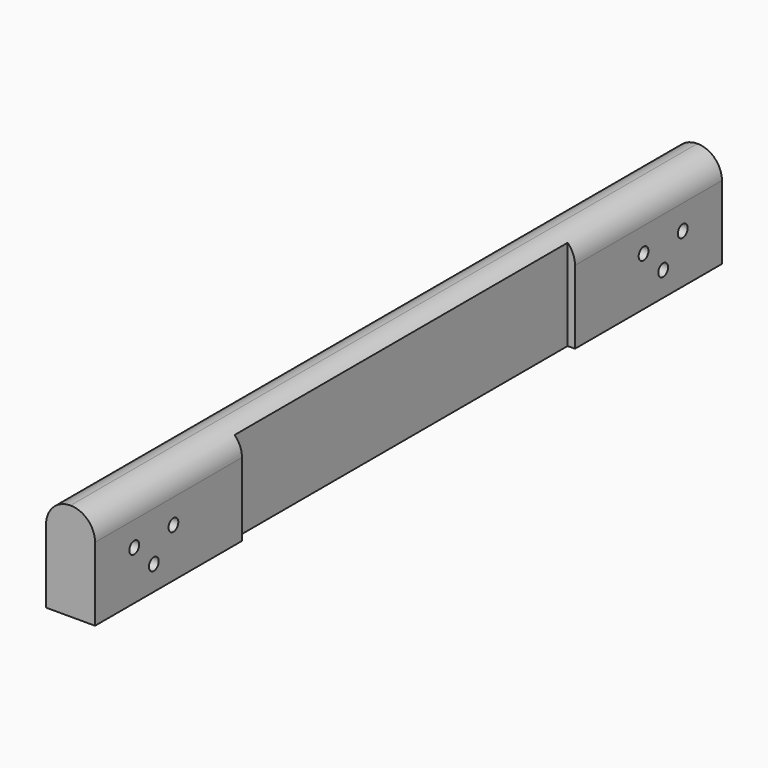
from build123d import *

# Parameters (mm, degrees)
F0_W     = 12.7
F0_H     = 25.4
F1_DEPTH = 101.6
F2_R     = 6.34999
F3_R     = 1.5875
F4_DEPTH = 25.4
F5_W     = 3.81
F5_H     = 107.95
F6_DEPTH = 25.4


# Not quite as in the source:
# - a fillet or chamfer is up to 0.001 mm smaller than in the source, because OpenCascade refuses the exact size


with BuildPart() as f1:
    # F0 (on Front) → F1 (new body, symmetric)
    with BuildSketch(Plane.XZ):
        Rectangle(F0_W, F0_H)
    extrude(amount=F1_DEPTH, both=True)

    # F2 (radius 6.35 in the source; OpenCascade refuses exactly that, so slightly less here)
    f2_edges = [f1.edges().sort_by_distance(p)[0] for p in [
        (-6.35, 0, 12.7),
        (6.35, 0, 12.7),
    ]]
    fillet(f2_edges, radius=F2_R)

    # F3 (on face) → F4 (cut)
    with BuildSketch(Plane(origin=(-6.35, 0, 0), x_dir=(0, -1, 0), z_dir=(-1, 0, 0))):
        with BuildLine():
            Line((-77.7875, 0), (-74.6125, 0))
            ThreePointArc((-74.6125, 0), (-76.2, 1.5875), (-77.7875, 0))
        make_face()
        with Locations((-88.9, 0)):
            Circle(F3_R)
        with BuildLine():
            ThreePointArc((90.4875, 0), (88.9, 1.5875), (87.3125, 0))
            ThreePointArc((87.3125, 0), (88.9, -1.5875), (90.4875, 0))
        make_face()
        with BuildLine():
            ThreePointArc((77.7875, 0), (76.2, 1.5875), (74.6125, 0))
            Line((74.6125, 0), (77.7875, 0))
        make_face()
        with BuildLine():
            Line((77.7875, 0), (74.6125, 0))
            ThreePointArc((74.6125, 0), (76.2, -1.5875), (77.7875, 0))
        make_face()
        with BuildLine():
            ThreePointArc((-77.7875, 0), (-76.2, -1.5875), (-74.6125, 0))
            Line((-74.6125, 0), (-77.7875, 0))
        make_face()
        with Locations((-82.55, -6.35)):
            Circle(F3_R)
        with Locations((82.55, -6.35)):
            Circle(F3_R)
    extrude(amount=-F4_DEPTH, mode=Mode.SUBTRACT)

    # F5 (on face) → F6 (cut)
    with BuildSketch(Plane(origin=(0, 0, -12.7), x_dir=(1, 0, 0), z_dir=(0, 0, -1))):
        with Locations((6.35, 0)):
            Rectangle(F5_W, F5_H)
    extrude(amount=-F6_DEPTH, mode=Mode.SUBTRACT)


solid = f1.part
